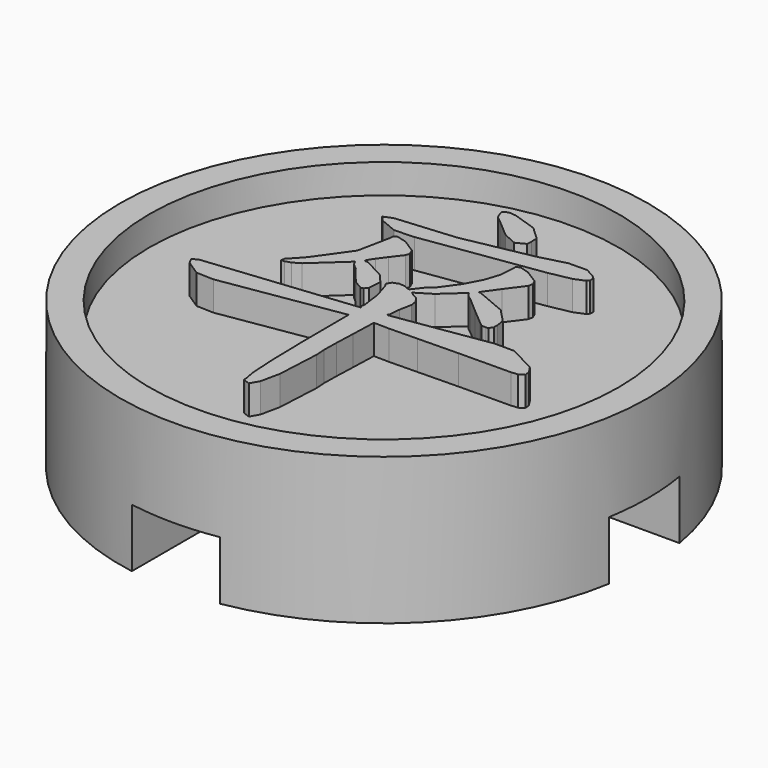
from build123d import *

# Parameters (mm, degrees)
F0_R     = 9
F1_DEPTH = 4
F3_W     = 3
F3_H     = 3
F4_DEPTH = 2
F2_R     = 9
F2_R_2   = 8
F5_DEPTH = 1
F7_DEPTH = 1


# Not quite as in the source:
# - a feature names something its author has since deleted; it is built from what else it names


with BuildPart() as f1:
    # F0 (on Top) → F1 (new body)
    with BuildSketch(Plane.XY):
        with Locations((-31.3306450844, 19.7580661625)):
            Circle(F0_R)
    extrude(amount=F1_DEPTH)

    # F3 (on face) → F4 (cut)
    with BuildSketch(Plane(origin=(0, 0, 0), x_dir=(1, 0, 0), z_dir=(0, 0, -1))):
        with BuildLine():
            ThreePointArc((-32.8306450844, -28.6321858371), (-32.0832814269, -28.7265408676), (-31.3306450844, -28.7580661625))
            ThreePointArc((-31.3306450844, -28.7580661625), (-30.5780087419, -28.7265408676), (-29.8306450844, -28.6321858371))
            Line((-29.8306450844, -28.6321858371), (-29.8306450844, -21.2580661625))
            Line((-29.8306450844, -21.2580661625), (-32.8306450844, -21.2580661625))
            Line((-32.8306450844, -21.2580661625), (-32.8306450844, -28.6321858371))
        make_face()
        with BuildLine():
            ThreePointArc((-40.204764759, -18.2580661625), (-40.2991197895, -19.0054298199), (-40.3306450844, -19.7580661625))
            ThreePointArc((-40.3306450844, -19.7580661625), (-40.2991197895, -20.510702505), (-40.204764759, -21.2580661625))
            Line((-40.204764759, -21.2580661625), (-32.8306450844, -21.2580661625))
            Line((-32.8306450844, -21.2580661625), (-32.8306450844, -18.2580661625))
            Line((-32.8306450844, -18.2580661625), (-40.204764759, -18.2580661625))
        make_face()
        with Locations((-31.3306450844, -19.7580661625)):
            Rectangle(F3_W, F3_H)
        with BuildLine():
            Line((-29.8306450844, -18.2580661625), (-29.8306450844, -21.2580661625))
            Line((-29.8306450844, -21.2580661625), (-22.4565254097, -21.2580661625))
            ThreePointArc((-22.4565254097, -21.2580661625), (-22.3621703793, -20.510702505), (-22.3306450844, -19.7580661625))
            ThreePointArc((-22.3306450844, -19.7580661625), (-22.3621703793, -19.0054298199), (-22.4565254097, -18.2580661625))
            Line((-22.4565254097, -18.2580661625), (-29.8306450844, -18.2580661625))
        make_face()
        with BuildLine():
            Line((-32.8306450844, -10.8839464878), (-32.8306450844, -18.2580661625))
            Line((-32.8306450844, -18.2580661625), (-29.8306450844, -18.2580661625))
            Line((-29.8306450844, -18.2580661625), (-29.8306450844, -10.8839464878))
            ThreePointArc((-29.8306450844, -10.8839464878), (-30.5780087419, -10.7895914574), (-31.3306450844, -10.7580661625))
            ThreePointArc((-31.3306450844, -10.7580661625), (-32.0832814269, -10.7895914574), (-32.8306450844, -10.8839464878))
        make_face()
    extrude(amount=-F4_DEPTH, mode=Mode.SUBTRACT)

    # F2 (on face) → F5 (join)
    with BuildSketch(Plane.XY.offset(4)):
        with Locations((-31.3306450844, 19.7580661625)):
            Circle(F2_R)
        with Locations((-31.3306450844, 19.7580661625)):
            Circle(F2_R_2, mode=Mode.SUBTRACT)
    extrude(amount=F5_DEPTH)

    # F6 (on face) → F7 (join)
    with BuildSketch(Plane.XY.offset(4)):
        Polygon((-31.9784342899, 25.4181322135), (-31.7774611038, 25.2590085979), (-31.1892692607, 24.7560993929), (-30.7208457687, 24.5338144768), (-30.4025390075, 24.6978790801), (-30.392716562, 24.8693254), (-30.4025390075, 25.1047664399), (-30.8471683696, 25.5198689359), (-31.6626039755, 25.7905517194), (-31.8783703596, 25.8094227206), (-32.0071634544, 25.7774551255), (-32.085100094, 25.7093528374), (-32.0432445706, 25.5871378045), align=None)
        Polygon((-32.0727952488, 23.82088353), (-34.1039519464, 23.641281604), (-34.4009291186, 23.5190665711), (-34.2549080498, 23.3492275605), (-33.6609834704, 23.1039640751), (-32.9981350893, 23.1326575217), (-28.9325058746, 23.7331363511), (-28.1966558885, 23.8783299532), (-27.8397737053, 24.0251903945), (-27.7799460833, 24.1039485477), (-27.774171676, 24.2417604333), (-27.925973105, 24.373024022), (-28.2204678774, 24.520658353), (-28.8430918564, 24.514110056), (-29.7462805942, 24.2778355965), align=None)
        Polygon((-34.382885584, 20.0842467066), (-33.3393966077, 21.0391074603), (-33.2631029954, 20.8914731293), (-33.073613141, 20.7339568229), (-32.8504769463, 20.4394620505), (-32.5781154176, 20.1235960182), (-32.2860792331, 19.9595314149), (-32.1999334103, 19.9800692553), (-32.1088704119, 20.0842467066), (-32.0826236472, 20.5436395019), (-32.3664685075, 20.8693279796), (-33.0604867821, 21.2294247813), (-33.1507282669, 21.2310916205), (-33.1753379574, 21.255677499), (-33.1457872792, 21.3246132068), (-33.0227447798, 21.5075488113), (-32.8135564575, 21.7938284475), (-32.5256159351, 22.1711889411), (-32.4854153449, 22.3016191102), (-32.5649890587, 22.4894957023), (-33.0170120434, 22.7807163262), (-33.3525229666, 22.866856196), (-33.4591649588, 22.8061356243), (-33.4673741419, 22.6765388749), (-33.689688823, 21.578925248), (-34.4845925415, 20.4550589033), (-34.7323443797, 20.1843165898), (-34.9046181661, 20.0087627019), (-34.9333294717, 19.8783325328), (-34.8291579734, 19.8807732617), (-34.6355486449, 19.9373862652), align=None)
        Polygon((-35.6429326931, 17.8857095862), (-31.560897018, 18.5354375615), (-31.5518663213, 16.6232038893), (-31.5215238944, 15.2286190431), (-31.4698399726, 14.3401836183), (-31.3968205087, 13.9447772089), (-31.3992731436, 13.8832511968), (-31.3443150733, 13.8561793466), (-31.1671300641, 13.7905517194), (-31.0005771079, 14.0834147752), (-30.8619318027, 14.7323117121), (-30.786507328, 16.2089407659), (-30.8094263673, 16.546904324), (-30.8012707611, 17.064559103), (-30.775851463, 17.7519993157), (-30.7470984864, 18.5977892544), (-30.2294853783, 18.5887585576), (-29.2737316751, 18.6067961392), (-27.8980535481, 18.6330488569), (-26.120369519, 18.6502887368), (-25.8890360471, 18.6707849062), (-25.726578753, 18.7749742635), (-25.7462831738, 18.9521771317), (-25.8939175048, 19.1818616234), (-26.8102623665, 19.6675071364), (-27.4952737563, 19.6675071364), (-28.9505434561, 19.4410967932), (-30.7340018925, 19.1687352645), (-30.7569209318, 19.1884337323), (-30.7208457687, 19.2343670588), (-30.6872113344, 19.6199188766), (-30.6060124524, 20.0350154196), (-30.6355393186, 20.2318810376), (-30.7602546103, 20.4156500617), (-30.9349750786, 20.502623351), (-31.0391525299, 20.5928707888), (-30.5207060022, 20.9111775501), (-29.8480173166, 21.5214788248), (-29.7602701377, 21.3886079269), (-29.5789418424, 21.255677499), (-29.0776994767, 20.8209301122), (-28.5387151086, 20.3664187747), (-28.4132259273, 20.2647415822), (-28.2466610651, 20.2515854584), (-28.17201048, 20.2655750018), (-28.0924784372, 20.3893973439), (-28.0924784372, 20.5501877988), (-28.1318277488, 20.8225374215), (-28.5707422337, 21.2827636364), (-29.618291154, 21.7249522697), (-29.6593073048, 21.7101888366), (-29.6707965895, 21.7249522697), (-29.2992105032, 22.2466729458), (-28.8668443153, 22.8275068844), (-28.8373174491, 22.9825229319), (-28.9062531568, 23.1457541156), (-29.3689201006, 23.4369747395), (-29.6937751587, 23.5296629062), (-29.8111087339, 23.461620148), (-29.8086084751, 23.3262489912), (-29.8455765878, 22.8619152083), (-30.0095816611, 22.3566248045), (-30.3074101119, 21.8037104229), (-30.7470984864, 21.1933496182), (-30.9267599424, 21.0588118811), (-31.2163375391, 20.6847255359), (-31.342677999, 20.7191933898), (-31.419793125, 20.7602095406), (-31.620772264, 20.7790805418), (-31.8135600789, 20.7077041052), (-31.9062541986, 20.5534619473), (-31.8398127967, 20.4419027794), (-31.6757303344, 19.9152411156), (-31.5871497358, 19.2474934177), (-31.6084674188, 19.1621869676), (-31.5740233769, 19.067010448), (-36.6470354491, 18.5354375615), (-36.8504809149, 18.4361653799), (-36.7356315255, 18.2302750181), (-36.2385062527, 17.9037709798), align=None)
    extrude(amount=F7_DEPTH)


solid = f1.part
